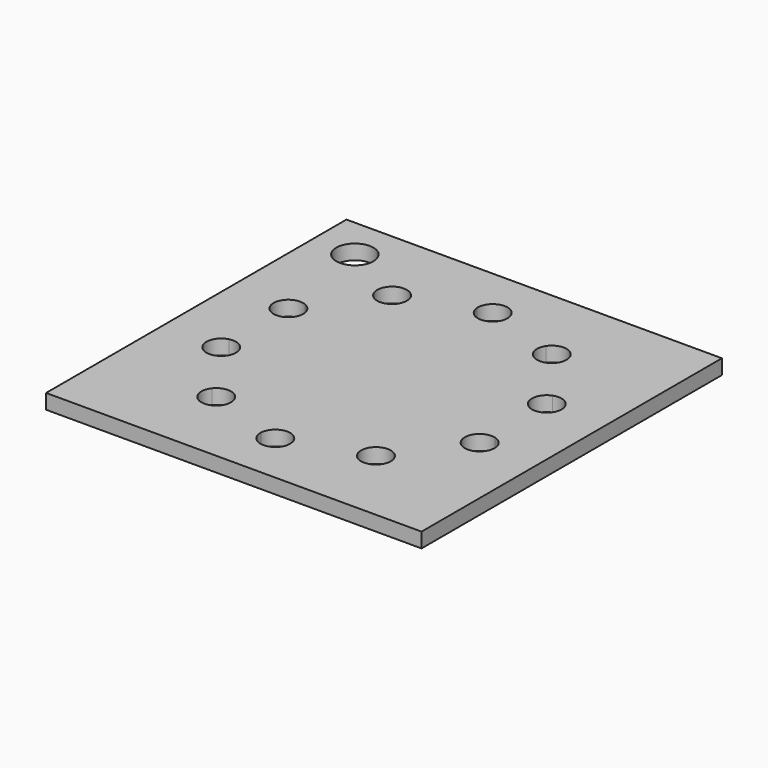
from build123d import *

# Parameters (mm, degrees)
F0_W     = 76
F0_H     = 76
F1_DEPTH = 3
F3_DEPTH = 25
F4_R     = 3.75
F5_DEPTH = 25


with BuildPart() as f1:
    # F0 (on Top) → F1 (new body)
    with BuildSketch(Plane.XY):
        Rectangle(F0_W, F0_H)
    extrude(amount=F1_DEPTH)

    # F2 (on face) → F3 (cut)
    with BuildSketch(Plane.XY.offset(3)):
        with BuildLine():
            ThreePointArc((25.0727558965, 11.2963229308), (23.3008846492, 7.5709163622), (26.9240976399, 5.5984789253))
            ThreePointArc((26.9240976399, 5.5984789253), (26.1540541981, 8.4979673453), (25.0727558965, 11.2963229308))
        make_face()
        with BuildLine():
            ThreePointArc((25.0727558965, 11.2963229308), (26.1540541981, 8.4979673453), (26.9240976399, 5.5984789253))
            ThreePointArc((26.9240976399, 5.5984789253), (28.5320922892, 6.669051044), (29.1540541981, 8.4979673453))
            ThreePointArc((29.1540541981, 8.4979673453), (27.8505366022, 10.9722242949), (25.0727558965, 11.2963229308))
        make_face()
        with BuildLine():
            ThreePointArc((29.1540541981, -8.4979673453), (28.5320922892, -6.669051044), (26.9240976399, -5.5984789253))
            ThreePointArc((26.9240976399, -5.5984789253), (26.1540541981, -8.4979673453), (25.0727558965, -11.2963229308))
            ThreePointArc((25.0727558965, -11.2963229308), (27.8505366022, -10.9722242949), (29.1540541981, -8.4979673453))
        make_face()
        with BuildLine():
            ThreePointArc((25.0727558965, -11.2963229308), (26.1540541981, -8.4979673453), (26.9240976399, -5.5984789253))
            ThreePointArc((26.9240976399, -5.5984789253), (23.3008846492, -7.5709163622), (25.0727558965, -11.2963229308))
        make_face()
        with BuildLine():
            ThreePointArc((13.6444735922, 23.8763133752), (14.4007386812, 19.8209163622), (18.4913492013, 20.3548521172))
            ThreePointArc((18.4913492013, 20.3548521172), (16.164094438, 22.2479673453), (13.6444735922, 23.8763133752))
        make_face()
        with BuildLine():
            ThreePointArc((13.6444735922, 23.8763133752), (16.164094438, 22.2479673453), (18.4913492013, 20.3548521172))
            ThreePointArc((18.4913492013, 20.3548521172), (18.990909279, 21.2434187626), (19.164094438, 22.2479673453))
            ThreePointArc((19.164094438, 22.2479673453), (17.0129576374, 25.1253674337), (13.6444735922, 23.8763133752))
        make_face()
        with BuildLine():
            ThreePointArc((19.164094438, -22.2479673453), (18.990909279, -21.2434187626), (18.4913492013, -20.3548521172))
            ThreePointArc((18.4913492013, -20.3548521172), (16.164094438, -22.2479673453), (13.6444735922, -23.8763133752))
            ThreePointArc((13.6444735922, -23.8763133752), (17.0129576374, -25.1253674337), (19.164094438, -22.2479673453))
        make_face()
        with BuildLine():
            ThreePointArc((13.6444735922, -23.8763133752), (16.164094438, -22.2479673453), (18.4913492013, -20.3548521172))
            ThreePointArc((18.4913492013, -20.3548521172), (14.4007386812, -19.8209163622), (13.6444735922, -23.8763133752))
        make_face()
        with BuildLine():
            ThreePointArc((-2.9955338657, 27.3363636364), (0, 24.5), (2.9955338657, 27.3363636364))
            ThreePointArc((2.9955338657, 27.3363636364), (0, 27.5), (-2.9955338657, 27.3363636364))
        make_face()
        with BuildLine():
            ThreePointArc((-2.9955338657, 27.3363636364), (0, 27.5), (2.9955338657, 27.3363636364))
            ThreePointArc((2.9955338657, 27.3363636364), (2.9988832586, 27.4181513503), (3, 27.5))
            ThreePointArc((3, 27.5), (-0.0818486497, 30.4988832586), (-2.9955338657, 27.3363636364))
        make_face()
        with BuildLine():
            ThreePointArc((3, -27.5), (2.9988832586, -27.4181513503), (2.9955338657, -27.3363636364))
            ThreePointArc((2.9955338657, -27.3363636364), (0, -27.5), (-2.9955338657, -27.3363636364))
            ThreePointArc((-2.9955338657, -27.3363636364), (-0.0818486497, -30.4988832586), (3, -27.5))
        make_face()
        with BuildLine():
            ThreePointArc((-2.9955338657, -27.3363636364), (0, -27.5), (2.9955338657, -27.3363636364))
            ThreePointArc((2.9955338657, -27.3363636364), (0, -24.5), (-2.9955338657, -27.3363636364))
        make_face()
        with BuildLine():
            ThreePointArc((-13.164094438, 22.2479673453), (-13.2866943496, 23.0968305447), (-13.6444735922, 23.8763133752))
            ThreePointArc((-13.6444735922, 23.8763133752), (-16.164094438, 22.2479673453), (-18.4913492013, 20.3548521172))
            ThreePointArc((-18.4913492013, 20.3548521172), (-15.1595458553, 19.4211525044), (-13.164094438, 22.2479673453))
        make_face()
        with BuildLine():
            ThreePointArc((-18.4913492013, 20.3548521172), (-16.164094438, 22.2479673453), (-13.6444735922, 23.8763133752))
            ThreePointArc((-13.6444735922, 23.8763133752), (-17.9274501949, 24.6750183284), (-18.4913492013, 20.3548521172))
        make_face()
        with BuildLine():
            ThreePointArc((-18.4913492013, -20.3548521172), (-17.9274501949, -24.6750183284), (-13.6444735922, -23.8763133752))
            ThreePointArc((-13.6444735922, -23.8763133752), (-16.164094438, -22.2479673453), (-18.4913492013, -20.3548521172))
        make_face()
        with BuildLine():
            ThreePointArc((-18.4913492013, -20.3548521172), (-16.164094438, -22.2479673453), (-13.6444735922, -23.8763133752))
            ThreePointArc((-13.6444735922, -23.8763133752), (-13.2866943496, -23.0968305447), (-13.164094438, -22.2479673453))
            ThreePointArc((-13.164094438, -22.2479673453), (-15.1595458553, -19.4211525044), (-18.4913492013, -20.3548521172))
        make_face()
        with BuildLine():
            ThreePointArc((-23.1540541981, 8.4979673453), (-23.6797972485, 10.1944497494), (-25.0727558965, 11.2963229308))
            ThreePointArc((-25.0727558965, 11.2963229308), (-26.1540541981, 8.4979673453), (-26.9240976399, 5.5984789253))
            ThreePointArc((-26.9240976399, 5.5984789253), (-24.3251378968, 6.1199292542), (-23.1540541981, 8.4979673453))
        make_face()
        with BuildLine():
            ThreePointArc((-26.9240976399, 5.5984789253), (-26.1540541981, 8.4979673453), (-25.0727558965, 11.2963229308))
            ThreePointArc((-25.0727558965, 11.2963229308), (-29.007223747, 9.4250183284), (-26.9240976399, 5.5984789253))
        make_face()
        with BuildLine():
            ThreePointArc((-26.9240976399, -5.5984789253), (-29.007223747, -9.4250183284), (-25.0727558965, -11.2963229308))
            ThreePointArc((-25.0727558965, -11.2963229308), (-26.1540541981, -8.4979673453), (-26.9240976399, -5.5984789253))
        make_face()
        with BuildLine():
            ThreePointArc((-26.9240976399, -5.5984789253), (-26.1540541981, -8.4979673453), (-25.0727558965, -11.2963229308))
            ThreePointArc((-25.0727558965, -11.2963229308), (-23.6797972485, -10.1944497494), (-23.1540541981, -8.4979673453))
            ThreePointArc((-23.1540541981, -8.4979673453), (-24.3251378968, -6.1199292542), (-26.9240976399, -5.5984789253))
        make_face()
    extrude(amount=-F3_DEPTH, mode=Mode.SUBTRACT)

    # F4 (on face) → F5 (cut)
    with BuildSketch(Plane.XY.offset(3)):
        with Locations((-29.5, 29.5)):
            Circle(F4_R)
    extrude(amount=-F5_DEPTH, mode=Mode.SUBTRACT)


solid = f1.part
